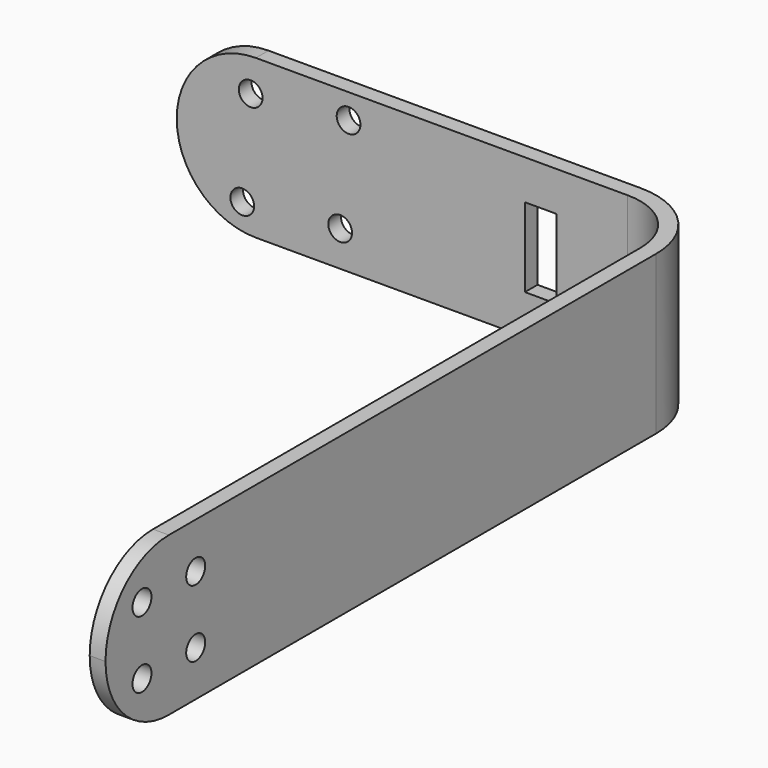
from build123d import *

# Parameters (mm, degrees)
F1_DEPTH = 20
F4_R     = 9.99999
F6_D     = 3
F2_W     = 4
F2_H     = 10
F7_DEPTH = 25
F8_D     = 3


# Not quite as in the source:
# - a fillet or chamfer is up to 0.001 mm smaller than in the source, because OpenCascade refuses the exact size
# - a feature names something its author has since deleted; it is built from what else it names


with BuildPart() as f1:
    # F0 (on Top) → F1 (new body)
    with BuildSketch(Plane.XY):
        with BuildLine():
            Line((0, 2), (0, 0))
            Line((0, 0), (57, 0))
            ThreePointArc((57, 0), (62.6568542495, -2.3431457505), (65, -8))
            Line((65, -8), (65, -95))
            Line((65, -95), (67, -95))
            Line((67, -95), (67, -8))
            ThreePointArc((67, -8), (64.0710678119, -0.9289321881), (57, 2))
            Line((57, 2), (0, 2))
        make_face()
    extrude(amount=F1_DEPTH)

    # F4 (radius 10 in the source; OpenCascade refuses exactly that, so slightly less here)
    f4_edges = [f1.edges().sort_by_distance(p)[0] for p in [
        (0, 1, 20),
        (0, 1, 0),
        (66, -95, 20),
        (66, -95, 0),
    ]]
    fillet(f4_edges, radius=F4_R)

    # F6 (through all)
    with Locations(Plane(origin=(65, 0, 0), x_dir=(0, -1, 0), z_dir=(-1, 0, 0))):
        with Locations((80.7573593129, 14.2426406871), (80.7573593129, 5.7573593129), (89.2426406871, 5.7573593129), (89.2426406871, 14.2426406871)):
            Hole(F6_D / 2)

    # F2 (on face) → F7 (cut)
    with BuildSketch(Plane.XZ):
        with Locations((46, 10)):
            Rectangle(F2_W, F2_H)
    extrude(amount=-F7_DEPTH, mode=Mode.SUBTRACT)

    # F8 (through all)
    with Locations(Plane.XZ):
        with Locations((8.2824855787, 3.4264645687), (21.7175144213, 16.8614934112), (20.6568542495, 4.4871247404), (9.3431457505, 15.8008332394)):
            Hole(F8_D / 2)


solid = f1.part
